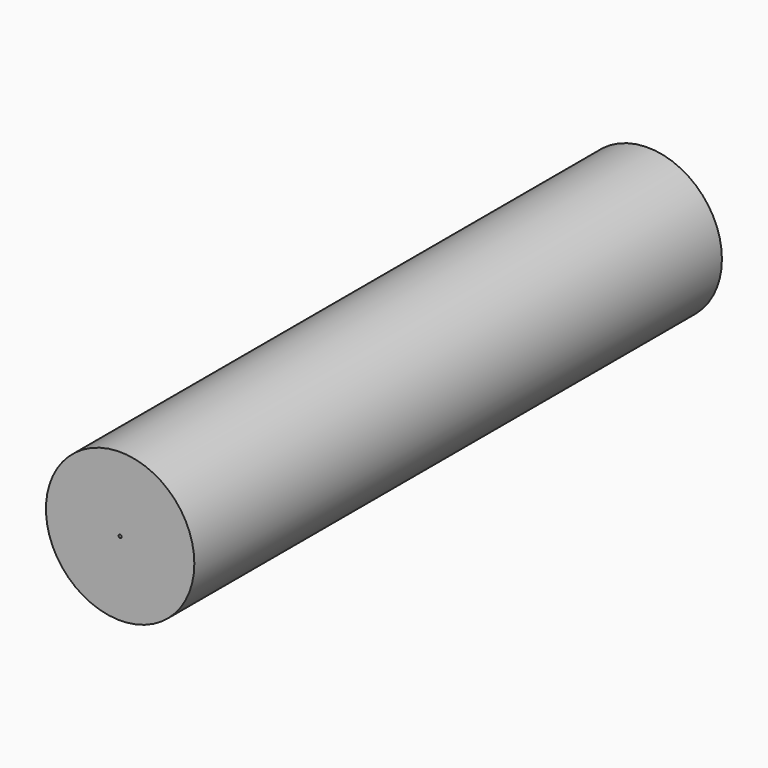
from build123d import *

# Parameters (mm, degrees)
F3_R     = 73.1333738811
F3_R_2   = 1.50312906
F4_DEPTH = 650


# Not quite as in the source:
# - the program builds the solid bodies; features that only make, move or delete a surface that nothing else refers to are left out


with BuildPart() as f4:
    # F3 (on Front) → F4 (new body)
    with BuildSketch(Plane.XZ):
        Circle(F3_R)
        Circle(F3_R_2, mode=Mode.SUBTRACT)
    extrude(amount=F4_DEPTH)


solid = f4.part
